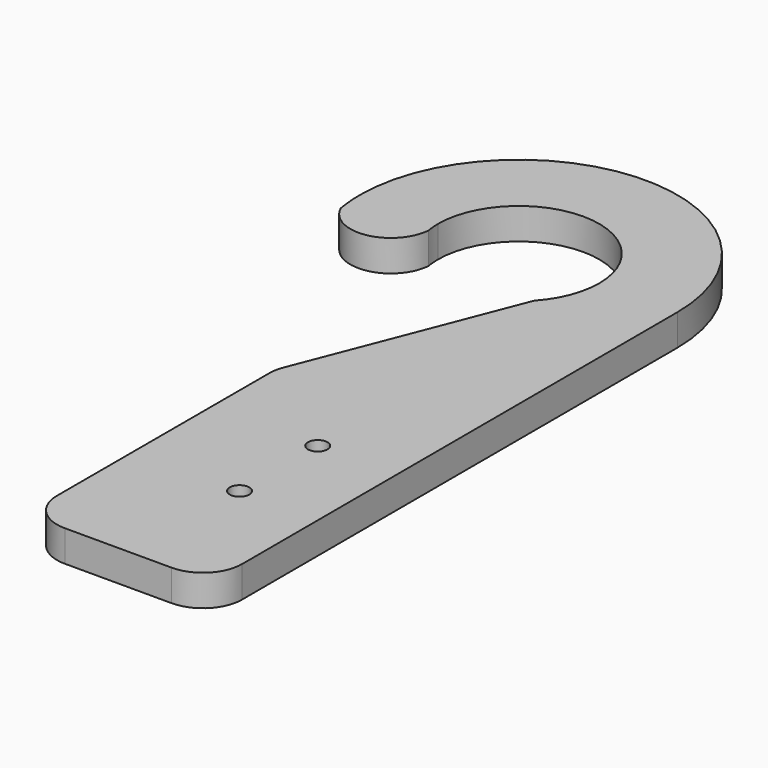
from build123d import *

# Parameters (mm, degrees)
F0_R     = 1.25
F1_DEPTH = 4
F2_R     = 5
F3_R     = 5
F4_R     = 5


# Not quite as in the source:
# - ends of sketch curves that miss each other by under 0.0002 mm in the source are joined


with BuildPart() as f1:
    # F0 (on Top) → F1 (new body)
    with BuildSketch(Plane.XY):
        with BuildLine():
            ThreePointArc((-20.6, 0), (-10.3, 10.3), (0, 0))
            ThreePointArc((0, 0), (-0.7054288039, -3.746225242), (-2.7250880706, -6.9793057865))
            Line((-2.7250880706, -6.9793057865), (-7.8691552748, -20.1539324679))
            ThreePointArc((-7.8691552748, -20.1539324679), (4.8894066362, -13.467439476), (10, 0))
            ThreePointArc((10, 0), (-10.3, 20.3), (-30.6, 0))
            ThreePointArc((-30.6, 0), (-25.6, 3.8602209978), (-20.6, 0))
        make_face()
        with BuildLine():
            ThreePointArc((-20.4505253001, -1.748381003), (-20.5625632907, -0.8773794529), (-20.6, 0))
            ThreePointArc((-20.6, 0), (-25.6, 3.8602209978), (-30.6, 0))
            ThreePointArc((-30.6, 0), (-30.526216971, -1.7292041645), (-30.3054042323, -3.4458382874))
            ThreePointArc((-30.3054042323, -3.4458382874), (-24.722708741, -6.4013107037), (-20.4505253001, -1.748381003))
        make_face()
        with BuildLine():
            ThreePointArc((10, 0), (4.8894066362, -13.467439476), (-7.8691552748, -20.1539324679))
            Line((-7.8691552748, -20.1539324679), (-13.5885840282, -34.8021350801))
            Line((-13.5885840282, -34.8021350801), (-13.5885840282, -74.6936649084))
            Line((-13.5885840282, -74.6936649084), (10.083315894, -74.6936649084))
            Line((10.083315894, -74.6936649084), (10, 0))
        make_face()
        with Locations((0, -57.5)):
            Circle(F0_R, mode=Mode.SUBTRACT)
        with Locations((0, -45)):
            Circle(F0_R, mode=Mode.SUBTRACT)
    extrude(amount=F1_DEPTH)

    # F2
    f2_edges = [f1.edges().sort_by_distance(p)[0] for p in [
        (-13.588584, -74.693665, 2),
    ]]
    fillet(f2_edges, radius=F2_R)

    # F3
    f3_edges = [f1.edges().sort_by_distance(p)[0] for p in [
        (10.083316, -74.693665, 2),
    ]]
    fillet(f3_edges, radius=F3_R)

    # F4
    f4_edges = [f1.edges().sort_by_distance(p)[0] for p in [
        (-13.588584, -34.802135, 2),
    ]]
    fillet(f4_edges, radius=F4_R)


solid = f1.part
